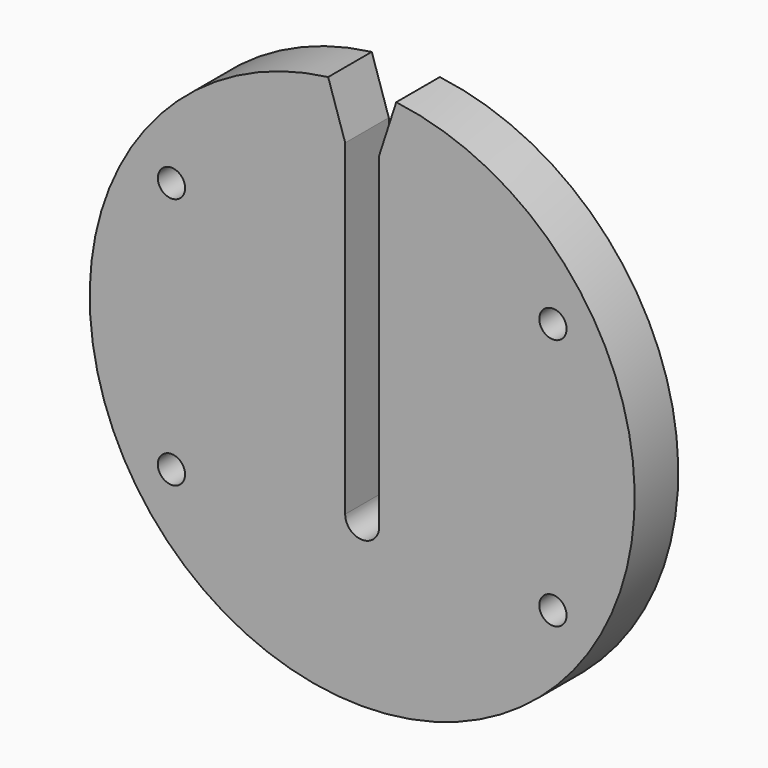
from build123d import *

# Parameters (mm, degrees)
F0_R           = 63.5
F1_DEPTH       = 12.7
F3_DEPTH       = 25.4
F4_D           = 6.35
F4_CBORE_D     = 10.3124
F4_CBORE_DEPTH = 6.35


# Not quite as in the source:
# - a feature names something its author has since deleted; it is built from what else it names


with BuildPart() as f1:
    # F0 (on Front) → F1 (new body)
    with BuildSketch(Plane.XZ):
        Circle(F0_R)
    extrude(amount=F1_DEPTH)

    # F2 (on face) → F3 (cut)
    with BuildSketch(Plane.XZ.offset(12.7)):
        with BuildLine():
            Line((-7.93115, 63.0027527944), (-3.96875, 50.8))
            Line((-3.96875, 50.8), (-3.96875, -25.4))
            ThreePointArc((-3.96875, -25.4), (0, -29.36875), (3.96875, -25.4))
            Line((3.96875, -25.4), (3.96875, 50.8))
            Line((3.96875, 50.8), (7.93115, 63.0027527944))
            ThreePointArc((7.93115, 63.0027527944), (0, 63.5), (-7.93115, 63.0027527944))
        make_face()
    extrude(amount=-F3_DEPTH, mode=Mode.SUBTRACT)

    # F4 (through all)
    with Locations(Plane(origin=(0, 0, 0), x_dir=(1, 0, 0), z_dir=(0, 1, 0))):
        with Locations((44.45, -29.36875), (-44.45, -29.36875), (44.45, 29.36875), (-44.45, 29.36875)):
            CounterBoreHole(F4_D / 2, F4_CBORE_D / 2, F4_CBORE_DEPTH)


solid = f1.part
